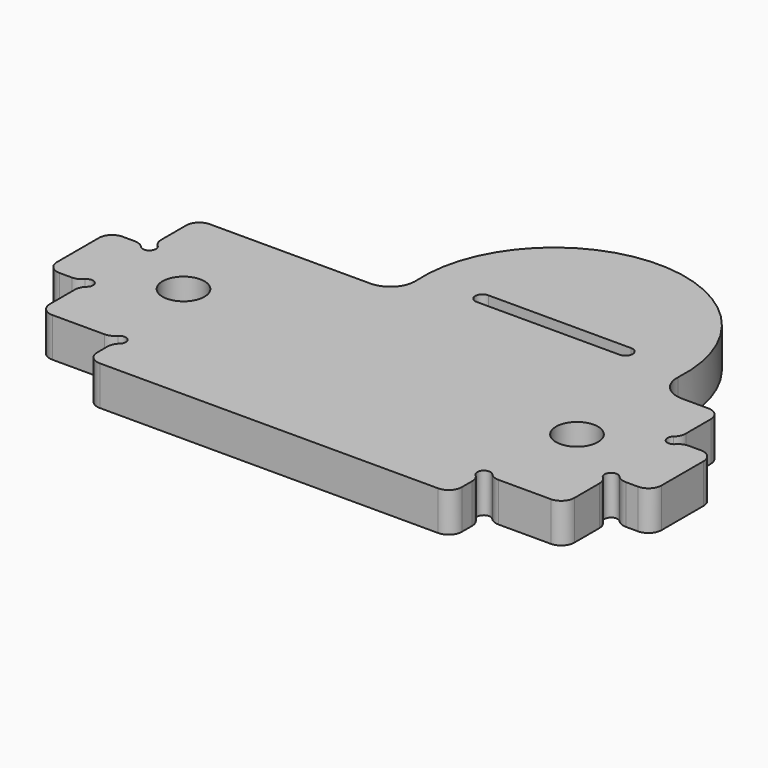
from build123d import *

# Parameters (mm, degrees)
F0_R     = 1.6
F1_DEPTH = 3
F2_W     = 3.05
F2_H     = 6
F3_DEPTH = 3
F5_D     = 1
F6_R     = 1


with BuildPart() as f1:
    # F0 (on Top) → F1 (new body)
    with BuildSketch(Plane.XY):
        with BuildLine():
            Line((-20, 0), (-20, -7.5))
            Line((-20, -7.5), (-13.9, -7.5))
            Line((-13.9, -7.5), (-13.9, -10.6))
            Line((-13.9, -10.6), (13.9, -10.6))
            Line((13.9, -10.6), (13.9, -7.5))
            Line((13.9, -7.5), (20, -7.5))
            Line((20, -7.5), (20, 0))
            Line((20, 0), (20, 7.5))
            Line((20, 7.5), (17, 7.5))
            ThreePointArc((17, 7.5), (15.615651922, 8.0992038794), (15.1050482082, 9.5186223298))
            ThreePointArc((15.1050482082, 9.5186223298), (5.125, 20.15), (-4.8550482082, 9.5186223298))
            ThreePointArc((-4.8550482082, 9.5186223298), (-5.365651922, 8.0992038794), (-6.75, 7.5))
            Line((-6.75, 7.5), (-20, 7.5))
            Line((-20, 7.5), (-20, 0))
        make_face()
        with Locations((-15, 0)):
            Circle(F0_R, mode=Mode.SUBTRACT)
        with Locations((15, 0)):
            Circle(F0_R, mode=Mode.SUBTRACT)
        with BuildLine():
            ThreePointArc((-0.325, 9.6), (-0.875, 10.15), (-0.325, 10.7))
            Line((-0.325, 10.7), (10.575, 10.7))
            ThreePointArc((10.575, 10.7), (10.9639087297, 10.5389087297), (11.125, 10.15))
            ThreePointArc((11.125, 10.15), (10.9639087297, 9.7610912703), (10.575, 9.6))
            Line((10.575, 9.6), (-0.325, 9.6))
        make_face(mode=Mode.SUBTRACT)
    extrude(amount=F1_DEPTH)

    # F2 (on face) → F3 (join, through all)
    with BuildSketch(Plane.XY.offset(3)):
        with Locations((-21.525, 0)):
            Rectangle(F2_W, F2_H)
        with Locations((21.525, 0)):
            Rectangle(F2_W, F2_H)
    extrude(amount=-F3_DEPTH)

    # F5 (through all)
    with Locations(Plane.XY.offset(3)):
        with Locations((13.9, -7.5), (20, -3), (20, 3), (-13.9, -7.5), (-20, -3), (-20, 3)):
            Hole(F5_D / 2)

    # F6
    f6_edges = [f1.edges().sort_by_distance(p)[0] for p in [
        (20, 7.5, 1.5),
        (23.05, 3, 1.5),
        (23.05, -3, 1.5),
        (13.9, -10.6, 1.5),
        (20, -7.5, 1.5),
        (-23.05, 3, 1.5),
        (-20, 7.5, 1.5),
        (-20, -7.5, 1.5),
        (-13.9, -10.6, 1.5),
        (-23.05, -3, 1.5),
        (20, 3.5, 1.5),
        (20.5, 3, 1.5),
        (20.5, -3, 1.5),
        (20, -3.5, 1.5),
        (14.4, -7.5, 1.5),
        (13.9, -8, 1.5),
        (-13.9, -8, 1.5),
        (-14.4, -7.5, 1.5),
        (-20, -3.5, 1.5),
        (-20.5, -3, 1.5),
        (-20.5, 3, 1.5),
        (-20, 3.5, 1.5),
    ]]
    fillet(f6_edges, radius=F6_R)


solid = f1.part
